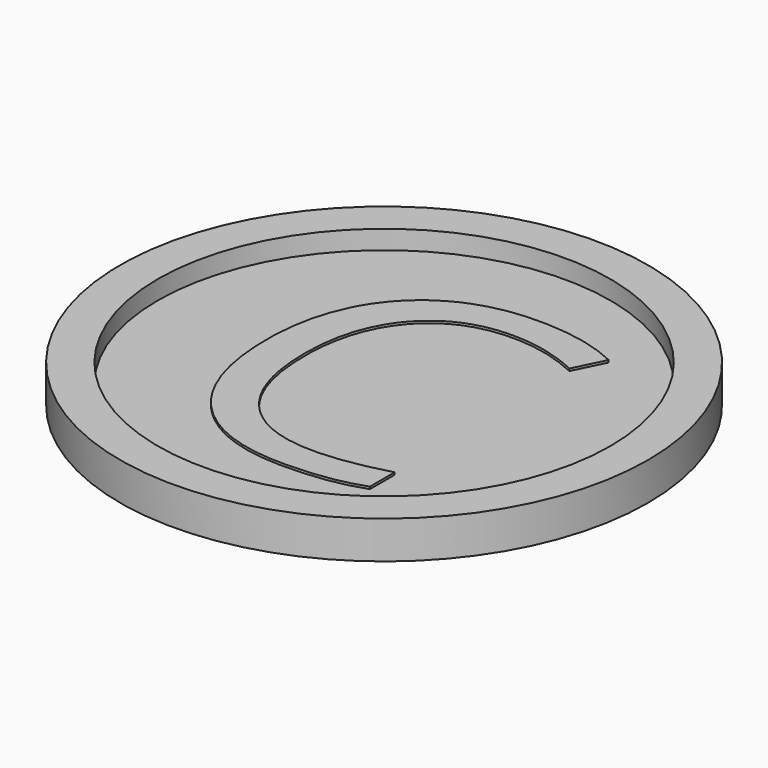
from build123d import *

# Parameters (mm, degrees)
F0_R         = 44.45
F1_DEPTH     = 6.35
F3_R         = 38.1
F4_DEPTH     = 3.175
F3_TEXT_SIZE = 71.8298812483
F5_DEPTH     = 2.794


# Not quite as in the source:
# - Text() gives the source's letters only with a copy of the font that has no kerning and outlines rounded to 1/6400 em; it was checked with that copy


with BuildPart() as f1:
    # F0 (on Top) → F1 (new body)
    with BuildSketch(Plane.XY):
        Circle(F0_R)
    extrude(amount=F1_DEPTH)

    # F3 (on offset) → F4 (cut)
    with BuildSketch(Plane.XY.offset(6.35)):
        Circle(F3_R)
        with BuildLine():
            add(Edge.make_bspline(
                [(16.7341176471, 18.0921513394), (10.9091632146, 20.8194421431), (5.0842087821, 20.8194421431)],
                knots=[0, 0, 0, 1, 1, 1], degree=2))
            add(Edge.make_bspline(
                [(5.0842087821, 20.8194421431), (-3.3670256835, 20.8194421431), (-8.2604363436, 15.1908975421)],
                knots=[0, 0, 0, 1, 1, 1], degree=2))
            add(Edge.make_bspline(
                [(-8.2604363436, 15.1908975421), (-13.1538470036, 9.5623529412), (-13.1538470036, -0.2244683789)],
                knots=[0, 0, 0, 1, 1, 1], degree=2))
            add(Edge.make_bspline(
                [(-13.1538470036, -0.2244683789), (-13.1538470036, -10.2806517537), (-8.4343993372, -15.7745153273)],
                knots=[0, 0, 0, 1, 1, 1], degree=2))
            add(Edge.make_bspline(
                [(-8.4343993372, -15.7745153273), (-3.7149516708, -21.2683789009), (5.0168682684, -21.2683789009)],
                knots=[0, 0, 0, 1, 1, 1], degree=2))
            add(Edge.make_bspline(
                [(5.0168682684, -21.2683789009), (10.3816625242, -21.2683789009), (17.2616183375, -19.3379508423)],
                knots=[0, 0, 0, 1, 1, 1], degree=2))
            Line((17.2616183375, -19.3379508423), (17.2616183375, -24.5568406518))
            add(Edge.make_bspline(
                [(17.2616183375, -24.5568406518), (11.9304943386, -26.5658326429), (4.1077713339, -26.5658326429)],
                knots=[0, 0, 0, 1, 1, 1], degree=2))
            add(Edge.make_bspline(
                [(4.1077713339, -26.5658326429), (-7.2166583817, -26.5658326429), (-13.372703673, -19.6858768296)],
                knots=[0, 0, 0, 1, 1, 1], degree=2))
            add(Edge.make_bspline(
                [(-13.372703673, -19.6858768296), (-19.5287489644, -12.8059210163), (-19.5287489644, -0.1459044463)],
                knots=[0, 0, 0, 1, 1, 1], degree=2))
            add(Edge.make_bspline(
                [(-19.5287489644, -0.1459044463), (-19.5287489644, 7.7778293289), (-16.5657663629, 13.7374647887)],
                knots=[0, 0, 0, 1, 1, 1], degree=2))
            add(Edge.make_bspline(
                [(-16.5657663629, 13.7374647887), (-13.6027837614, 19.6971002486), (-8.0079094173, 22.9238331952)],
                knots=[0, 0, 0, 1, 1, 1], degree=2))
            add(Edge.make_bspline(
                [(-8.0079094173, 22.9238331952), (-2.4130350732, 26.1505661419), (5.1627727147, 26.1505661419)],
                knots=[0, 0, 0, 1, 1, 1], degree=2))
            add(Edge.make_bspline(
                [(5.1627727147, 26.1505661419), (13.2211875173, 26.1505661419), (19.2593869097, 23.2100303783)],
                knots=[0, 0, 0, 1, 1, 1], degree=2))
            Line((19.2593869097, 23.2100303783), (16.7341176471, 18.0921513394))
        make_face(mode=Mode.SUBTRACT)
    extrude(amount=-F4_DEPTH, mode=Mode.SUBTRACT)

    # F3 (on offset) → F5 (cut)
    with BuildSketch(Plane.XY.offset(6.35)):
        with Locations((-23.9171057719, -25.8587572494)):
            Text('C', F3_TEXT_SIZE, font='Open Sans', text_align=(TextAlign.LEFT, TextAlign.BOTTOM))
    extrude(amount=-F5_DEPTH, mode=Mode.SUBTRACT)


solid = f1.part
